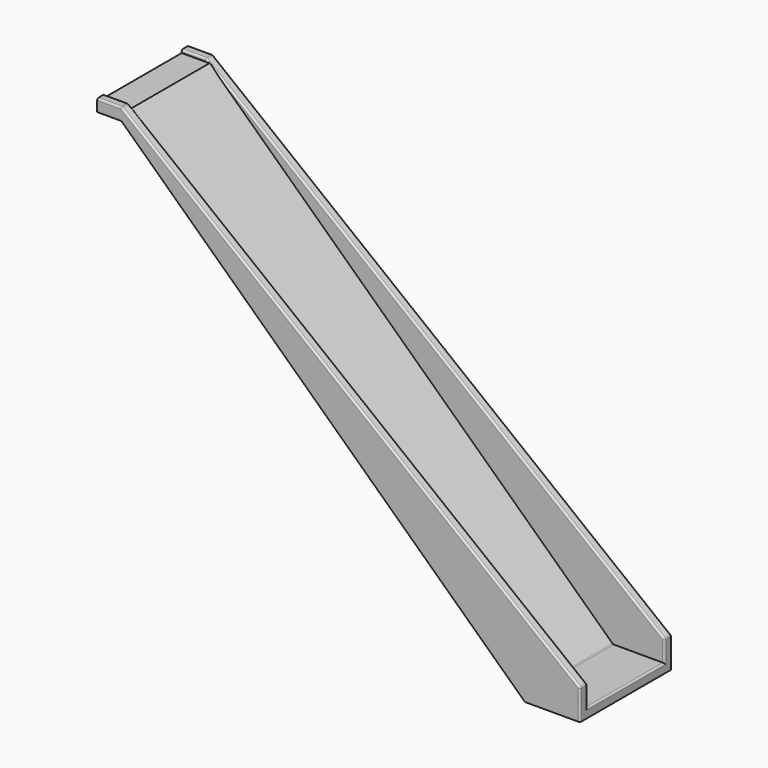
from build123d import *

# Parameters (mm, degrees)
F1_DEPTH      = 482.6
F2_T          = -38.1
F3_T1_DEPTH   = 421.5195451874
F3_T3_DEPTH   = 118.0046220681
F3_T5_DEPTH   = 2453.1375416599
F3_T7_DEPTH   = 22.86
F3_T9_DEPTH   = 22.86
F3_T11_DEPTH  = 142.3573332117
F3_T13_DEPTH  = 85.2073332117
F3_T15_DEPTH  = 406.4
F3_T20_DEPTH  = 7.7724
F3_T26_DEPTH  = 7.7724
F3_T32_DEPTH  = 7.7724
F3_T38_DEPTH  = 7.7724
F3_T44_DEPTH  = 7.7724
F3_T50_DEPTH  = 7.7724
F3_T56_DEPTH  = 7.7724
F3_T62_DEPTH  = 7.7724
F3_T68_DEPTH  = 2453.1375416599
F3_T73_DEPTH  = 2453.1375416599
F3_T78_DEPTH  = 2453.1375416599
F3_T83_DEPTH  = 2453.1375416599
F3_T89_DEPTH  = 104.2573332117
F3_T93_DEPTH  = 425.45
F3_T100_DEPTH = 104.2573332117
F3_T104_DEPTH = 425.45


# Not quite as in the source:
# - a fillet or chamfer that OpenCascade refuses, or shapes differently, is made with other operations: its cross-section is extruded or revolved along the edge and cut away or added


with BuildPart() as f1:
    # F0 (on Front) → F1 (new body)
    with BuildSketch(Plane.XZ):
        Polygon((-1698.6751983284, 1600.2), (0, 0), (231.7248016716, 0), (231.7248016716, 127), (-1698.6751983284, 1651), (-1800.2751983284, 1651), (-1800.2751983284, 1600.2), align=None)
    extrude(amount=F1_DEPTH)

    # F2
    f2_openings = [f1.faces().sort_by_distance(p)[0] for p in [
        (-733.475198, -241.3, 889),
        (231.724802, -241.3, 63.5),
        (-1749.475198, -241.3, 1651),
        (-1800.275198, -241.3, 1625.6),
    ]]
    offset(amount=F2_T, openings=f2_openings, kind=Kind.INTERSECTION)

    # F3: fillet of radius 7.62 on 18 edges, made by hand

    # F3_s2 → F3_t1 (join)
    with BuildSketch(Plane.XZ.offset(30.5402274063)):
        with BuildLine():
            ThreePointArc((12.918470552, 40.1734744552), (15.3327714476, 38.6373124927), (18.1434542249, 38.1))
            Line((18.1434542249, 38.1), (15.1195451874, 38.1))
            Line((15.1195451874, 38.1), (12.918470552, 40.1734744552))
        make_face()
    extrude(amount=F3_T1_DEPTH)

    # F3_s4 → F3_t3 (cut)
    with BuildSketch(Plane.YZ.offset(-1819.3251983284)):
        with BuildLine():
            ThreePointArc((-444.5, 1643.38), (-446.7318463274, 1648.7681536726), (-452.12, 1651))
            Line((-452.12, 1651), (-444.5, 1651))
            Line((-444.5, 1651), (-444.5, 1643.38))
        make_face()
        with BuildLine():
            ThreePointArc((-482.6, 1643.38), (-480.3681536726, 1648.7681536726), (-474.98, 1651))
            Line((-474.98, 1651), (-482.6, 1651))
            Line((-482.6, 1651), (-482.6, 1643.38))
        make_face()
        with BuildLine():
            ThreePointArc((-30.48, 1651), (-35.8681536726, 1648.7681536726), (-38.1, 1643.38))
            Line((-38.1, 1643.38), (-38.1, 1651))
            Line((-38.1, 1651), (-30.48, 1651))
        make_face()
        with BuildLine():
            ThreePointArc((0, 1643.38), (-2.2318463274, 1648.7681536726), (-7.62, 1651))
            Line((-7.62, 1651), (0, 1651))
            Line((0, 1651), (0, 1643.38))
        make_face()
    extrude(amount=F3_T3_DEPTH, mode=Mode.SUBTRACT)

    # F3_s6 → F3_t5 (cut)
    with BuildSketch(Plane(origin=(78.0874461401, 0, -61.6479837949), x_dir=(0, 1, 0), z_dir=(-0.7848827655, 0, 0.6196442886))):
        with BuildLine():
            ThreePointArc((-482.6, -235.6470611007), (-480.3681536726, -241.0352147733), (-474.98, -243.2670611007))
            Line((-474.98, -243.2670611007), (-482.6, -243.2670611007))
            Line((-482.6, -243.2670611007), (-482.6, -235.6470611007))
        make_face()
        with BuildLine():
            ThreePointArc((0, -235.6470611007), (-2.2318463274, -241.0352147733), (-7.62, -243.2670611007))
            Line((-7.62, -243.2670611007), (0, -243.2670611007))
            Line((0, -243.2670611007), (0, -235.6470611007))
        make_face()
    extrude(amount=F3_T5_DEPTH, mode=Mode.SUBTRACT)

    # F3_s8 → F3_t7 (cut)
    with BuildSketch(Plane.XZ.offset(7.62)):
        with BuildLine():
            ThreePointArc((-1701.3205762603, 1651), (-1698.8215111202, 1650.578546619), (-1696.5988867813, 1649.3608066734))
            Line((-1696.5988867813, 1649.3608066734), (-1698.6751983284, 1651))
            Line((-1698.6751983284, 1651), (-1701.3205762603, 1651))
        make_face()
        with BuildLine():
            ThreePointArc((231.7248016716, 123.3073332117), (230.9620487078, 126.6303684334), (228.8264911506, 129.288139885))
            Line((228.8264911506, 129.288139885), (231.7248016716, 127))
            Line((231.7248016716, 127), (231.7248016716, 123.3073332117))
        make_face()
    extrude(amount=F3_T7_DEPTH, mode=Mode.SUBTRACT)

    # F3_s10 → F3_t9 (cut)
    with BuildSketch(Plane.XZ.offset(452.12)):
        with BuildLine():
            ThreePointArc((-1701.3205762603, 1651), (-1698.8215111202, 1650.578546619), (-1696.5988867813, 1649.3608066734))
            Line((-1696.5988867813, 1649.3608066734), (-1698.6751983284, 1651))
            Line((-1698.6751983284, 1651), (-1701.3205762603, 1651))
        make_face()
        with BuildLine():
            ThreePointArc((231.7248016716, 123.3073332117), (230.9620487078, 126.6303684334), (228.8264911506, 129.288139885))
            Line((228.8264911506, 129.288139885), (231.7248016716, 127))
            Line((231.7248016716, 127), (231.7248016716, 123.3073332117))
        make_face()
    extrude(amount=F3_T9_DEPTH, mode=Mode.SUBTRACT)

    # F3_s12 → F3_t11 (cut)
    with BuildSketch(Plane.XY.offset(-19.05)):
        with BuildLine():
            ThreePointArc((224.1048016716, -482.6), (229.4929553442, -480.3681536726), (231.7248016716, -474.98))
            Line((231.7248016716, -474.98), (231.7248016716, -482.6))
            Line((231.7248016716, -482.6), (224.1048016716, -482.6))
        make_face()
        with BuildLine():
            ThreePointArc((224.1048016716, 0), (229.4929553442, -2.2318463274), (231.7248016716, -7.62))
            Line((231.7248016716, -7.62), (231.7248016716, 0))
            Line((231.7248016716, 0), (224.1048016716, 0))
        make_face()
    extrude(amount=F3_T11_DEPTH, mode=Mode.SUBTRACT)

    # F3_s14 → F3_t13 (cut)
    with BuildSketch(Plane.XY.offset(38.1)):
        with BuildLine():
            ThreePointArc((224.1048016716, -38.1), (229.4929553442, -35.8681536726), (231.7248016716, -30.48))
            Line((231.7248016716, -30.48), (231.7248016716, -38.1))
            Line((231.7248016716, -38.1), (224.1048016716, -38.1))
        make_face()
        with BuildLine():
            ThreePointArc((224.1048016716, -444.5), (229.4929553442, -446.7318463274), (231.7248016716, -452.12))
            Line((231.7248016716, -452.12), (231.7248016716, -444.5))
            Line((231.7248016716, -444.5), (224.1048016716, -444.5))
        make_face()
    extrude(amount=F3_T13_DEPTH, mode=Mode.SUBTRACT)

    # F3_s16 → F3_t15 (cut)
    with BuildSketch(Plane.XZ.offset(38.1)):
        with BuildLine():
            ThreePointArc((231.7248016716, 30.48), (229.4929553442, 35.8681536726), (224.1048016716, 38.1))
            Line((224.1048016716, 38.1), (231.7248016716, 38.1))
            Line((231.7248016716, 38.1), (231.7248016716, 30.48))
        make_face()
    extrude(amount=F3_T15_DEPTH, mode=Mode.SUBTRACT)


with BuildPart() as f3_tool18:
    # F3_s19 → F3_t20 (new body)
    with BuildSketch(Plane.XZ.offset(452.12)):
        Polygon((-1701.3205762603, 1643.38), (-1701.3205762603, 1651.1524), (-1698.6222907698, 1651.1524), (-1696.5044529917, 1649.4804228068), align=None)
    extrude(amount=-F3_T20_DEPTH)

    # F3_s21 → F3_t22 (revolve, cut)
    with BuildSketch(Plane(origin=(-1701.3205762603, -452.12, 1643.38), x_dir=(-0.3279613045, 0, -0.9446911573), z_dir=(0.9446911573, 0, -0.3279613045))):
        with BuildLine():
            ThreePointArc((0, -7.62), (7.62, 0), (0, 7.62))
            Line((0, 7.62), (0, -7.62))
        make_face()
    revolve(axis=Axis((-1701.3205762603, -452.12, 1643.38), (0, 1, 0)), mode=Mode.SUBTRACT)


with BuildPart() as f1_1:
    add(f1.part)

    # F3_t17: cut F3_tool18
    add(f3_tool18.part, mode=Mode.SUBTRACT)


with BuildPart() as f3_tool24:
    # F3_s25 → F3_t26 (new body)
    with BuildSketch(Plane.XZ.offset(452.12)):
        Polygon((224.1048016716, 123.3073332117), (231.8772016716, 123.3073332117), (231.8772016716, 127.0738533358), (228.9209249402, 129.4077560185), align=None)
    extrude(amount=-F3_T26_DEPTH)

    # F3_s27 → F3_t28 (revolve, cut)
    with BuildSketch(Plane(origin=(224.1048016716, -452.12, 123.3073332117), x_dir=(-0.8999011858, 0, -0.4360938611), z_dir=(0.4360938611, 0, -0.8999011858))):
        with BuildLine():
            ThreePointArc((0, -7.62), (7.62, 0), (0, 7.62))
            Line((0, 7.62), (0, -7.62))
        make_face()
    revolve(axis=Axis((224.1048016716, -452.12, 123.3073332117), (0, 1, 0)), mode=Mode.SUBTRACT)


with BuildPart() as f1_2:
    add(f1_1.part)

    # F3_t23: cut F3_tool24
    add(f3_tool24.part, mode=Mode.SUBTRACT)


with BuildPart() as f3_tool30:
    # F3_s31 → F3_t32 (new body)
    with BuildSketch(Plane.XZ.offset(474.98)):
        Polygon((-1701.3205762603, 1643.38), (-1696.5044529917, 1649.4804228068), (-1698.6222907698, 1651.1524), (-1701.3205762603, 1651.1524), align=None)
    extrude(amount=F3_T32_DEPTH)

    # F3_s33 → F3_t34 (revolve, cut)
    with BuildSketch(Plane(origin=(-1701.3205762603, -474.98, 1643.38), x_dir=(-0.3279613045, 0, -0.9446911573), z_dir=(-0.9446911573, 0, 0.3279613045))):
        with BuildLine():
            ThreePointArc((0, -7.62), (7.62, 0), (0, 7.62))
            Line((0, 7.62), (0, -7.62))
        make_face()
    revolve(axis=Axis((-1701.3205762603, -474.98, 1643.38), (0, -1, 0)), mode=Mode.SUBTRACT)


with BuildPart() as f1_3:
    add(f1_2.part)

    # F3_t29: cut F3_tool30
    add(f3_tool30.part, mode=Mode.SUBTRACT)


with BuildPart() as f3_tool36:
    # F3_s37 → F3_t38 (new body)
    with BuildSketch(Plane.XZ.offset(474.98)):
        Polygon((224.1048016716, 123.3073332117), (228.9209249402, 129.4077560185), (231.8772016716, 127.0738533358), (231.8772016716, 123.3073332117), align=None)
    extrude(amount=F3_T38_DEPTH)

    # F3_s39 → F3_t40 (revolve, cut)
    with BuildSketch(Plane(origin=(224.1048016716, -474.98, 123.3073332117), x_dir=(-0.8999011858, 0, -0.4360938611), z_dir=(-0.4360938611, 0, 0.8999011858))):
        with BuildLine():
            ThreePointArc((0, -7.62), (7.62, 0), (0, 7.62))
            Line((0, 7.62), (0, -7.62))
        make_face()
    revolve(axis=Axis((224.1048016716, -474.98, 123.3073332117), (0, -1, 0)), mode=Mode.SUBTRACT)


with BuildPart() as f1_4:
    add(f1_3.part)

    # F3_t35: cut F3_tool36
    add(f3_tool36.part, mode=Mode.SUBTRACT)


with BuildPart() as f3_tool42:
    # F3_s43 → F3_t44 (new body)
    with BuildSketch(Plane.XZ.offset(30.48)):
        Polygon((-1701.3205762603, 1643.38), (-1696.5044529917, 1649.4804228068), (-1698.6222907698, 1651.1524), (-1701.3205762603, 1651.1524), align=None)
    extrude(amount=F3_T44_DEPTH)

    # F3_s45 → F3_t46 (revolve, cut)
    with BuildSketch(Plane(origin=(-1701.3205762603, -30.48, 1643.38), x_dir=(-0.3279613045, 0, -0.9446911573), z_dir=(-0.9446911573, 0, 0.3279613045))):
        with BuildLine():
            ThreePointArc((0, -7.62), (7.62, 0), (0, 7.62))
            Line((0, 7.62), (0, -7.62))
        make_face()
    revolve(axis=Axis((-1701.3205762603, -30.48, 1643.38), (0, -1, 0)), mode=Mode.SUBTRACT)


with BuildPart() as f1_5:
    add(f1_4.part)

    # F3_t41: cut F3_tool42
    add(f3_tool42.part, mode=Mode.SUBTRACT)


with BuildPart() as f3_tool48:
    # F3_s49 → F3_t50 (new body)
    with BuildSketch(Plane.XZ.offset(7.62)):
        Polygon((-1701.3205762603, 1643.38), (-1696.5044529917, 1649.4804228068), (-1698.6222907698, 1651.1524), (-1701.3205762603, 1651.1524), align=None)
    extrude(amount=-F3_T50_DEPTH)

    # F3_s51 → F3_t52 (revolve, cut)
    with BuildSketch(Plane(origin=(-1701.3205762603, -7.62, 1643.38), x_dir=(-0.3279613045, 0, -0.9446911573), z_dir=(0.9446911573, 0, -0.3279613045))):
        with BuildLine():
            ThreePointArc((0, -7.62), (7.62, 0), (0, 7.62))
            Line((0, 7.62), (0, -7.62))
        make_face()
    revolve(axis=Axis((-1701.3205762603, -7.62, 1643.38), (0, 1, 0)), mode=Mode.SUBTRACT)


with BuildPart() as f1_6:
    add(f1_5.part)

    # F3_t47: cut F3_tool48
    add(f3_tool48.part, mode=Mode.SUBTRACT)


with BuildPart() as f3_tool54:
    # F3_s55 → F3_t56 (new body)
    with BuildSketch(Plane.XZ.offset(7.62)):
        Polygon((224.1048016716, 123.3073332117), (228.9209249402, 129.4077560185), (231.8772016716, 127.0738533358), (231.8772016716, 123.3073332117), align=None)
    extrude(amount=-F3_T56_DEPTH)

    # F3_s57 → F3_t58 (revolve, cut)
    with BuildSketch(Plane(origin=(224.1048016716, -7.62, 123.3073332117), x_dir=(-0.8999011858, 0, -0.4360938611), z_dir=(0.4360938611, 0, -0.8999011858))):
        with BuildLine():
            ThreePointArc((0, -7.62), (7.62, 0), (0, 7.62))
            Line((0, 7.62), (0, -7.62))
        make_face()
    revolve(axis=Axis((224.1048016716, -7.62, 123.3073332117), (0, 1, 0)), mode=Mode.SUBTRACT)


with BuildPart() as f1_7:
    add(f1_6.part)

    # F3_t53: cut F3_tool54
    add(f3_tool54.part, mode=Mode.SUBTRACT)


with BuildPart() as f3_tool60:
    # F3_s61 → F3_t62 (new body)
    with BuildSketch(Plane.XZ.offset(30.48)):
        Polygon((224.1048016716, 123.3073332117), (231.8772016716, 123.3073332117), (231.8772016716, 127.0738533358), (228.9209249402, 129.4077560185), align=None)
    extrude(amount=F3_T62_DEPTH)

    # F3_s63 → F3_t64 (revolve, cut)
    with BuildSketch(Plane(origin=(224.1048016716, -30.48, 123.3073332117), x_dir=(-0.8999011858, 0, -0.4360938611), z_dir=(-0.4360938611, 0, 0.8999011858))):
        with BuildLine():
            ThreePointArc((0, -7.62), (7.62, 0), (0, 7.62))
            Line((0, 7.62), (0, -7.62))
        make_face()
    revolve(axis=Axis((224.1048016716, -30.48, 123.3073332117), (0, -1, 0)), mode=Mode.SUBTRACT)


with BuildPart() as f1_8:
    add(f1_7.part)

    # F3_t59: cut F3_tool60
    add(f3_tool60.part, mode=Mode.SUBTRACT)


with BuildPart() as f3_tool66:
    # F3_s67 → F3_t68 (new body)
    with BuildSketch(Plane(origin=(78.0874461401, 0, -61.6479837949), x_dir=(0, 1, 0), z_dir=(-0.7848827655, 0, 0.6196442886))):
        with BuildLine():
            ThreePointArc((-444.5, -235.6470611007), (-446.7318463274, -241.0352147733), (-452.12, -243.2670611007))
            Line((-452.12, -243.2670611007), (-444.5, -243.2670611007))
            Line((-444.5, -243.2670611007), (-444.5, -235.6470611007))
        make_face()
    extrude(amount=F3_T68_DEPTH)

    split(bisect_by=Plane(origin=(26.1249183642, 0, 27.7326277238), x_dir=(0, 1, 0), z_dir=(0.6856933954, 0, 0.7278904914)), keep=Keep.TOP)


with BuildPart() as f1_9:
    add(f1_8.part)

    # F3_t65: cut F3_tool66
    add(f3_tool66.part, mode=Mode.SUBTRACT)


with BuildPart() as f3_tool71:
    # F3_s72 → F3_t73 (new body)
    with BuildSketch(Plane(origin=(78.0874461401, 0, -61.6479837949), x_dir=(0, 1, 0), z_dir=(-0.7848827655, 0, 0.6196442886))):
        with BuildLine():
            ThreePointArc((-444.5, -235.6470611007), (-446.7318463274, -241.0352147733), (-452.12, -243.2670611007))
            Line((-452.12, -243.2670611007), (-444.5, -243.2670611007))
            Line((-444.5, -243.2670611007), (-444.5, -235.6470611007))
        make_face()
    extrude(amount=F3_T73_DEPTH)

    split(bisect_by=Plane.XY.offset(1638.3), keep=Keep.TOP)


with BuildPart() as f1_10:
    add(f1_9.part)

    # F3_t70: cut F3_tool71
    add(f3_tool71.part, mode=Mode.SUBTRACT)


with BuildPart() as f3_tool76:
    # F3_s77 → F3_t78 (new body)
    with BuildSketch(Plane(origin=(78.0874461401, 0, -61.6479837949), x_dir=(0, 1, 0), z_dir=(-0.7848827655, 0, 0.6196442886))):
        with BuildLine():
            ThreePointArc((-38.1, -235.6470611007), (-35.8681536726, -241.0352147733), (-30.48, -243.2670611007))
            Line((-30.48, -243.2670611007), (-38.1, -243.2670611007))
            Line((-38.1, -243.2670611007), (-38.1, -235.6470611007))
        make_face()
    extrude(amount=F3_T78_DEPTH)

    split(bisect_by=Plane(origin=(26.1249183642, 0, 27.7326277238), x_dir=(0, 1, 0), z_dir=(0.6856933954, 0, 0.7278904914)), keep=Keep.TOP)


with BuildPart() as f1_11:
    add(f1_10.part)

    # F3_t75: cut F3_tool76
    add(f3_tool76.part, mode=Mode.SUBTRACT)


with BuildPart() as f3_tool81:
    # F3_s82 → F3_t83 (new body)
    with BuildSketch(Plane(origin=(78.0874461401, 0, -61.6479837949), x_dir=(0, 1, 0), z_dir=(-0.7848827655, 0, 0.6196442886))):
        with BuildLine():
            ThreePointArc((-38.1, -235.6470611007), (-35.8681536726, -241.0352147733), (-30.48, -243.2670611007))
            Line((-30.48, -243.2670611007), (-38.1, -243.2670611007))
            Line((-38.1, -243.2670611007), (-38.1, -235.6470611007))
        make_face()
    extrude(amount=F3_T83_DEPTH)

    split(bisect_by=Plane.XY.offset(1638.3), keep=Keep.TOP)


with BuildPart() as f1_12:
    add(f1_11.part)

    # F3_t80: cut F3_tool81
    add(f3_tool81.part, mode=Mode.SUBTRACT)


with BuildPart() as f3_tool87:
    # F3_s88 → F3_t89 (new body)
    with BuildSketch(Plane.XY.offset(19.05)):
        with BuildLine():
            ThreePointArc((224.1048016716, -38.1), (229.4929553442, -35.8681536726), (231.7248016716, -30.48))
            Line((231.7248016716, -30.48), (231.7248016716, -38.1))
            Line((231.7248016716, -38.1), (224.1048016716, -38.1))
        make_face()
    extrude(amount=F3_T89_DEPTH)

    split(bisect_by=Plane.XY.offset(38.1), keep=Keep.BOTTOM)


with BuildPart() as f3_tool91:
    # F3_s92 → F3_t93 (new body)
    with BuildSketch(Plane.XZ.offset(444.5)):
        with BuildLine():
            ThreePointArc((231.7248016716, 30.48), (229.4929553442, 35.8681536726), (224.1048016716, 38.1))
            Line((224.1048016716, 38.1), (231.7248016716, 38.1))
            Line((231.7248016716, 38.1), (231.7248016716, 30.48))
        make_face()
    extrude(amount=-F3_T93_DEPTH)

    split(bisect_by=Plane.XZ.offset(38.1), keep=Keep.BOTTOM)


with BuildPart() as f3_tool87_1:
    add(f3_tool87.part)

    # F3_t95: intersect F3_tool91
    add(f3_tool91.part, mode=Mode.INTERSECT)


with BuildPart() as f1_13:
    add(f1_12.part)

    # F3_t85: cut F3_tool87
    add(f3_tool87_1.part, mode=Mode.SUBTRACT)


with BuildPart() as f3_tool98:
    # F3_s99 → F3_t100 (new body)
    with BuildSketch(Plane.XY.offset(19.05)):
        with BuildLine():
            ThreePointArc((224.1048016716, -444.5), (229.4929553442, -446.7318463274), (231.7248016716, -452.12))
            Line((231.7248016716, -452.12), (231.7248016716, -444.5))
            Line((231.7248016716, -444.5), (224.1048016716, -444.5))
        make_face()
    extrude(amount=F3_T100_DEPTH)

    split(bisect_by=Plane.XY.offset(38.1), keep=Keep.BOTTOM)


with BuildPart() as f3_tool102:
    # F3_s103 → F3_t104 (new body)
    with BuildSketch(Plane.XZ.offset(463.55)):
        with BuildLine():
            ThreePointArc((231.7248016716, 30.48), (229.4929553442, 35.8681536726), (224.1048016716, 38.1))
            Line((224.1048016716, 38.1), (231.7248016716, 38.1))
            Line((231.7248016716, 38.1), (231.7248016716, 30.48))
        make_face()
    extrude(amount=-F3_T104_DEPTH)

    split(bisect_by=Plane.XZ.offset(444.5), keep=Keep.TOP)


with BuildPart() as f3_tool98_1:
    add(f3_tool98.part)

    # F3_t106: intersect F3_tool102
    add(f3_tool102.part, mode=Mode.INTERSECT)


with BuildPart() as f1_14:
    add(f1_13.part)

    # F3_t96: cut F3_tool98
    add(f3_tool98_1.part, mode=Mode.SUBTRACT)


solid = f1_14.part
